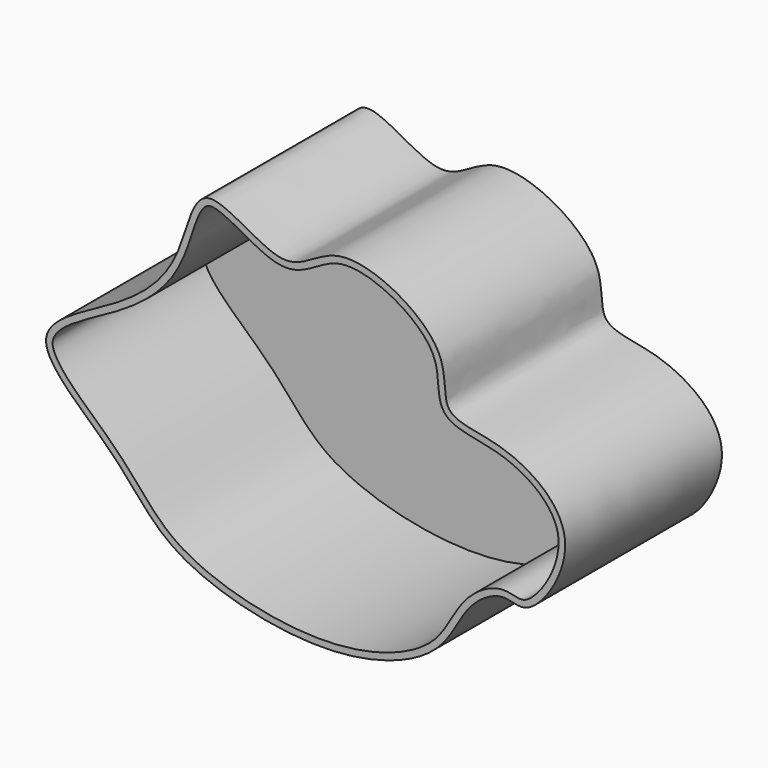
from build123d import *

# Parameters (mm, degrees)
F1_DEPTH = 76.2
F2_T     = -2.54


with BuildPart() as f1:
    # F0 (on Front) → F1 (new body)
    with BuildSketch(Plane.XZ):
        with BuildLine():
            add(Edge.make_bspline(
                [(41.7877584696, 52.3419901729), (44.8018027838, 48.2894034099), (64.4881749943, 48.8617228919), (97.1090820354, 25.6170049562), (73.6524525111, -10.5567415214), (62.6532135389, -2.6084169176), (47.1016330699, -12.4907392198), (39.8950198203, -34.5636019236), (-4.3647350441, -51.1089230817), (-68.8433379183, -34.9837775872), (-84.9792045589, -5.7751896586), (-129.7400412914, 26.8713959161), (-86.3002032434, 45.375556858), (-61.7932088079, 66.1817124447), (-56.8403586929, 106.430796245), (-20.6412690628, 73.191240814), (-2.2664490215, 100.382757886), (44.5541749084, 74.9110955698), (38.9685340092, 56.1326284445), (41.7877584696, 52.3419901729)],
                knots=[0, 0, 0, 0, 0.0505734858, 0.1130511893, 0.1734015489, 0.2067598716, 0.2489136506, 0.2988616417, 0.3702126757, 0.45515277, 0.5197965051, 0.5877261956, 0.6491909644, 0.7138346995, 0.7689926899, 0.8294744224, 0.8825031066, 0.9526954506, 1, 1, 1, 1], degree=3))
        make_face()
    extrude(amount=F1_DEPTH)

    # F2
    f2_openings = [f1.faces().sort_by_distance(p)[0] for p in [
        (-13.60377, -76.2, 21.839055),
    ]]
    offset(amount=F2_T, openings=f2_openings)


solid = f1.part
